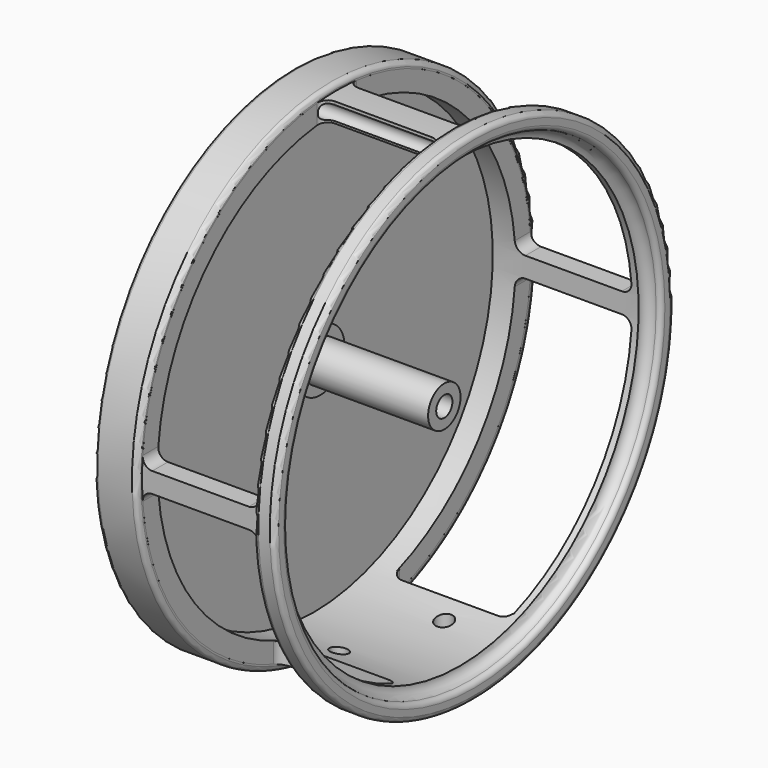
from build123d import *

# Parameters (mm, degrees)
F2_R      = 0.762
F3_DEPTH  = 5.08
F4_R      = 1.143
F5_DEPTH  = 22.225
F7_DEPTH  = 304.8
F9_DEPTH  = 44.45
F11_DEPTH = 50.8
F12_W     = 13.335
F12_H     = 2.54
F13_DEPTH = 12.7
F16_R     = 0.76199
F17_R     = 38.1
F17_R_2   = 3.175
F18_DEPTH = 1.524
F23_R     = 0.762
F24_R     = 1.1176
F25_DEPTH = 22.098
F27_D     = 2.7051


# Not quite as in the source:
# - a fillet or chamfer is up to 0.001 mm smaller than in the source, because OpenCascade refuses the exact size


with BuildPart() as f1:
    # F0 (on Front) → F1 (revolve)
    with BuildSketch(Plane.XZ):
        with BuildLine():
            Line((24.384, 38.1), (0, 38.1))
            Line((0, 38.1), (0, 35.052))
            Line((0, 35.052), (22.86, 35.052))
            ThreePointArc((22.86, 35.052), (23.3063692655, 36.1296307345), (24.384, 36.576))
            Line((24.384, 36.576), (24.384, 38.1))
        make_face()
    revolve(axis=Axis((27.4000445678, 0, 0), (1, 0, 0)))

    # F2 (on face) → F3 (cut)
    with BuildSketch(Plane(origin=(0, 0, 0), x_dir=(0, -1, 0), z_dir=(-1, 0, 0))):
        with Locations((0, 36.195)):
            Circle(F2_R)
        with Locations((-36.195, 0)):
            Circle(F2_R)
        with Locations((36.195, 0)):
            Circle(F2_R)
    extrude(amount=-F3_DEPTH, mode=Mode.SUBTRACT)

    # F4 (on Right) → F5 (cut)
    with BuildSketch(Plane.YZ):
        with Locations((2.5469832476, 36.4235573851)):
            Circle(F4_R)
        with Locations((-2.5469832476, 36.4235573851)):
            Circle(F4_R)
    extrude(amount=F5_DEPTH, mode=Mode.SUBTRACT)

    # F6 (on Top) → F7 (cut)
    with BuildSketch(Plane.XY):
        with BuildLine():
            ThreePointArc((5.1435, 2.286), (6.2660320151, 2.7509679849), (6.731, 3.8735))
            ThreePointArc((6.731, 3.8735), (5.1435, 5.461), (3.556, 3.8735))
            ThreePointArc((3.556, 3.8735), (4.0209679849, 2.7509679849), (5.1435, 2.286))
        make_face()
        with BuildLine():
            ThreePointArc((3.556, 3.8735), (5.1435, 5.461), (6.731, 3.8735))
            ThreePointArc((6.731, 3.8735), (6.2660320151, 2.7509679849), (5.1435, 2.286))
            Line((5.1435, 2.286), (20.2565, 2.286))
            ThreePointArc((20.2565, 2.286), (19.1339679849, 4.9960320151), (21.844, 3.8735))
            Line((21.844, 3.8735), (21.844, 31.8135))
            ThreePointArc((21.844, 31.8135), (19.1339679849, 30.6909679849), (20.2565, 33.401))
            Line((20.2565, 33.401), (5.1435, 33.401))
            ThreePointArc((5.1435, 33.401), (6.2660320151, 32.9360320151), (6.731, 31.8135))
            ThreePointArc((6.731, 31.8135), (5.1435, 30.226), (3.556, 31.8135))
            Line((3.556, 31.8135), (3.556, 3.8735))
        make_face()
        with BuildLine():
            ThreePointArc((5.1435, 33.401), (4.0209679849, 32.9360320151), (3.556, 31.8135))
            ThreePointArc((3.556, 31.8135), (5.1435, 30.226), (6.731, 31.8135))
            ThreePointArc((6.731, 31.8135), (6.2660320151, 32.9360320151), (5.1435, 33.401))
        make_face()
        with BuildLine():
            ThreePointArc((21.844, 3.8735), (19.1339679849, 4.9960320151), (20.2565, 2.286))
            ThreePointArc((20.2565, 2.286), (21.3790320151, 2.7509679849), (21.844, 3.8735))
        make_face()
        with BuildLine():
            ThreePointArc((21.844, 31.8135), (21.3790320151, 32.9360320151), (20.2565, 33.401))
            ThreePointArc((20.2565, 33.401), (19.1339679849, 30.6909679849), (21.844, 31.8135))
        make_face()
        with BuildLine():
            ThreePointArc((20.2565, -33.401), (21.3790320151, -32.9360320151), (21.844, -31.8135))
            ThreePointArc((21.844, -31.8135), (19.1339679849, -30.6909679849), (20.2565, -33.401))
        make_face()
        with BuildLine():
            ThreePointArc((20.2565, -33.401), (19.1339679849, -30.6909679849), (21.844, -31.8135))
            Line((21.844, -31.8135), (21.844, -3.8735))
            ThreePointArc((21.844, -3.8735), (19.1339679849, -4.9960320151), (20.2565, -2.286))
            Line((20.2565, -2.286), (5.1435, -2.286))
            ThreePointArc((5.1435, -2.286), (6.2660320151, -2.7509679849), (6.731, -3.8735))
            ThreePointArc((6.731, -3.8735), (5.1435, -5.461), (3.556, -3.8735))
            Line((3.556, -3.8735), (3.556, -31.8135))
            ThreePointArc((3.556, -31.8135), (5.1435, -30.226), (6.731, -31.8135))
            ThreePointArc((6.731, -31.8135), (6.2660320151, -32.9360320151), (5.1435, -33.401))
            Line((5.1435, -33.401), (20.2565, -33.401))
        make_face()
        with BuildLine():
            ThreePointArc((20.2565, -2.286), (19.1339679849, -4.9960320151), (21.844, -3.8735))
            ThreePointArc((21.844, -3.8735), (21.3790320151, -2.7509679849), (20.2565, -2.286))
        make_face()
        with BuildLine():
            ThreePointArc((3.556, -31.8135), (4.0209679849, -32.9360320151), (5.1435, -33.401))
            ThreePointArc((5.1435, -33.401), (6.2660320151, -32.9360320151), (6.731, -31.8135))
            ThreePointArc((6.731, -31.8135), (5.1435, -30.226), (3.556, -31.8135))
        make_face()
        with BuildLine():
            ThreePointArc((6.731, -3.8735), (6.2660320151, -2.7509679849), (5.1435, -2.286))
            ThreePointArc((5.1435, -2.286), (4.0209679849, -2.7509679849), (3.556, -3.8735))
            ThreePointArc((3.556, -3.8735), (5.1435, -5.461), (6.731, -3.8735))
        make_face()
    extrude(amount=F7_DEPTH, mode=Mode.SUBTRACT)

    # F8 (on Front) → F9 (cut, symmetric)
    with BuildSketch(Plane.XZ):
        with BuildLine():
            ThreePointArc((5.1435, 1.5875), (6.2660320151, 2.0524679849), (6.731, 3.175))
            ThreePointArc((6.731, 3.175), (5.1435, 4.7625), (3.556, 3.175))
            ThreePointArc((3.556, 3.175), (4.0209679849, 2.0524679849), (5.1435, 1.5875))
        make_face()
        with BuildLine():
            ThreePointArc((3.556, 3.175), (5.1435, 4.7625), (6.731, 3.175))
            ThreePointArc((6.731, 3.175), (6.2660320151, 2.0524679849), (5.1435, 1.5875))
            Line((5.1435, 1.5875), (20.2565, 1.5875))
            ThreePointArc((20.2565, 1.5875), (19.1339679849, 4.2975320151), (21.844, 3.175))
            Line((21.844, 3.175), (21.844, 33.02))
            Line((21.844, 33.02), (3.556, 33.02))
            Line((3.556, 33.02), (3.556, 3.175))
        make_face()
        with BuildLine():
            ThreePointArc((21.844, 3.175), (19.1339679849, 4.2975320151), (20.2565, 1.5875))
            ThreePointArc((20.2565, 1.5875), (21.3790320151, 2.0524679849), (21.844, 3.175))
        make_face()
        with BuildLine():
            Line((3.556, -33.02), (21.844, -33.02))
            Line((21.844, -33.02), (21.844, -3.175))
            ThreePointArc((21.844, -3.175), (19.1339679849, -4.2975320151), (20.2565, -1.5875))
            Line((20.2565, -1.5875), (5.1435, -1.5875))
            ThreePointArc((5.1435, -1.5875), (6.2660320151, -2.0524679849), (6.731, -3.175))
            ThreePointArc((6.731, -3.175), (5.1435, -4.7625), (3.556, -3.175))
            Line((3.556, -3.175), (3.556, -33.02))
        make_face()
        with BuildLine():
            ThreePointArc((20.2565, -1.5875), (19.1339679849, -4.2975320151), (21.844, -3.175))
            ThreePointArc((21.844, -3.175), (21.3790320151, -2.0524679849), (20.2565, -1.5875))
        make_face()
        with BuildLine():
            ThreePointArc((5.1435, -1.5875), (4.0209679849, -2.0524679849), (3.556, -3.175))
            ThreePointArc((3.556, -3.175), (5.1435, -4.7625), (6.731, -3.175))
            ThreePointArc((6.731, -3.175), (6.2660320151, -2.0524679849), (5.1435, -1.5875))
        make_face()
    extrude(amount=F9_DEPTH, both=True, mode=Mode.SUBTRACT)

    # F10 (on Top) → F11 (cut)
    with BuildSketch(Plane.XY):
        with BuildLine():
            ThreePointArc((5.1435, 10.795), (6.2660320151, 11.2599679849), (6.731, 12.3825))
            ThreePointArc((6.731, 12.3825), (5.1435, 13.97), (3.556, 12.3825))
            ThreePointArc((3.556, 12.3825), (4.0209679849, 11.2599679849), (5.1435, 10.795))
        make_face()
        with BuildLine():
            ThreePointArc((3.556, 12.3825), (5.1435, 13.97), (6.731, 12.3825))
            ThreePointArc((6.731, 12.3825), (6.2660320151, 11.2599679849), (5.1435, 10.795))
            Line((5.1435, 10.795), (20.2565, 10.795))
            ThreePointArc((20.2565, 10.795), (19.1339679849, 13.5050320151), (21.844, 12.3825))
            Line((21.844, 12.3825), (21.844, 33.401))
            Line((21.844, 33.401), (3.556, 33.401))
            Line((3.556, 33.401), (3.556, 12.3825))
        make_face()
        with BuildLine():
            ThreePointArc((21.844, 12.3825), (19.1339679849, 13.5050320151), (20.2565, 10.795))
            ThreePointArc((20.2565, 10.795), (21.3790320151, 11.2599679849), (21.844, 12.3825))
        make_face()
        with BuildLine():
            Line((20.2565, -10.795), (5.1435, -10.795))
            ThreePointArc((5.1435, -10.795), (6.2660320151, -11.2599679849), (6.731, -12.3825))
            ThreePointArc((6.731, -12.3825), (5.1435, -13.97), (3.556, -12.3825))
            Line((3.556, -12.3825), (3.556, -33.401))
            Line((3.556, -33.401), (21.844, -33.401))
            Line((21.844, -33.401), (21.844, -12.3825))
            ThreePointArc((21.844, -12.3825), (19.1339679849, -13.5050320151), (20.2565, -10.795))
        make_face()
        with BuildLine():
            ThreePointArc((6.731, -12.3825), (6.2660320151, -11.2599679849), (5.1435, -10.795))
            ThreePointArc((5.1435, -10.795), (4.0209679849, -11.2599679849), (3.556, -12.3825))
            ThreePointArc((3.556, -12.3825), (5.1435, -13.97), (6.731, -12.3825))
        make_face()
        with BuildLine():
            ThreePointArc((21.844, -12.3825), (21.3790320151, -11.2599679849), (20.2565, -10.795))
            ThreePointArc((20.2565, -10.795), (19.1339679849, -13.5050320151), (21.844, -12.3825))
        make_face()
    extrude(amount=-F11_DEPTH, mode=Mode.SUBTRACT)

    # F12 (on Front) → F13 (cut, symmetric)
    with BuildSketch(Plane.XZ):
        with Locations((12.192, -37.973)):
            Rectangle(F12_W, F12_H)
    extrude(amount=F13_DEPTH, both=True, mode=Mode.SUBTRACT)

    # F27 (through all)
    with Locations(Plane(origin=(0, 0, -36.703), x_dir=(1, 0, 0), z_dir=(0, 0, -1))):
        with Locations((9.652, 7.112), (14.732, -7.112)):
            Hole(F27_D / 2)


with BuildPart() as f15:
    # F14 (on Front) → F15 (revolve)
    with BuildSketch(Plane.XZ):
        Polygon((24.384, 38.1), (24.384, 36.576), (25.146, 36.576), (25.146, 39.116), (21.844, 39.116), (21.844, 38.1), align=None)
    revolve(axis=Axis((27.4000445678, 0, 0), (1, 0, 0)))

    # F16 (radius 0.762 in the source; OpenCascade refuses exactly that, so slightly less here)
    f16_edges = [f15.edges().sort_by_distance(p)[0] for p in [
        (25.146, 0, -36.576),
        (25.146, 0, -39.116),
        (21.844, 0, -39.116),
    ]]
    fillet(f16_edges, radius=F16_R)


with BuildPart() as f18:
    # F17 (on Right) → F18 (new body)
    with BuildSketch(Plane.YZ):
        Circle(F17_R)
        Circle(F17_R_2, mode=Mode.SUBTRACT)
    extrude(amount=-F18_DEPTH)


with BuildPart() as f20:
    # F19 (on Front) → F20 (revolve)
    with BuildSketch(Plane.XZ):
        Polygon((-1.524, 3.175), (-1.524, 1.5875), (20.447, 1.5875), (20.447, 3.175), (1.016, 3.175), (1.016, 4.7625), (0, 4.7625), (0, 3.175), align=None)
    revolve(axis=Axis((27.4000445678, 0, 0), (1, 0, 0)))


with BuildPart() as f22:
    # F21 (on Front) → F22 (revolve)
    with BuildSketch(Plane.XZ):
        with BuildLine():
            Line((-1.524, 38.1), (3.556, 38.1))
            Line((3.556, 38.1), (3.556, 39.116))
            Line((3.556, 39.116), (-2.54, 39.116))
            ThreePointArc((-2.54, 39.116), (-3.048, 38.608), (-2.54, 38.1))
            Line((-2.54, 38.1), (-2.54, 34.036))
            Line((-2.54, 34.036), (-1.524, 34.036))
            Line((-1.524, 34.036), (-1.524, 38.1))
        make_face()
    revolve(axis=Axis((27.4000445678, 0, 0), (1, 0, 0)))

    # F23
    f23_edges = [f22.edges().sort_by_distance(p)[0] for p in [
        (3.556, 0, -39.116),
        (-2.54, 0, -34.036),
    ]]
    fillet(f23_edges, radius=F23_R)


with BuildPart() as f25:
    # F24 (on face) → F25 (new body)
    with BuildSketch(Plane(origin=(0, 0, 0), x_dir=(0, -1, 0), z_dir=(-1, 0, 0))):
        with Locations((-2.5469832476, 36.4235573851)):
            Circle(F24_R)
    extrude(amount=-F25_DEPTH)


solid = Compound([f1.part, f15.part, f18.part, f20.part, f22.part, f25.part])
